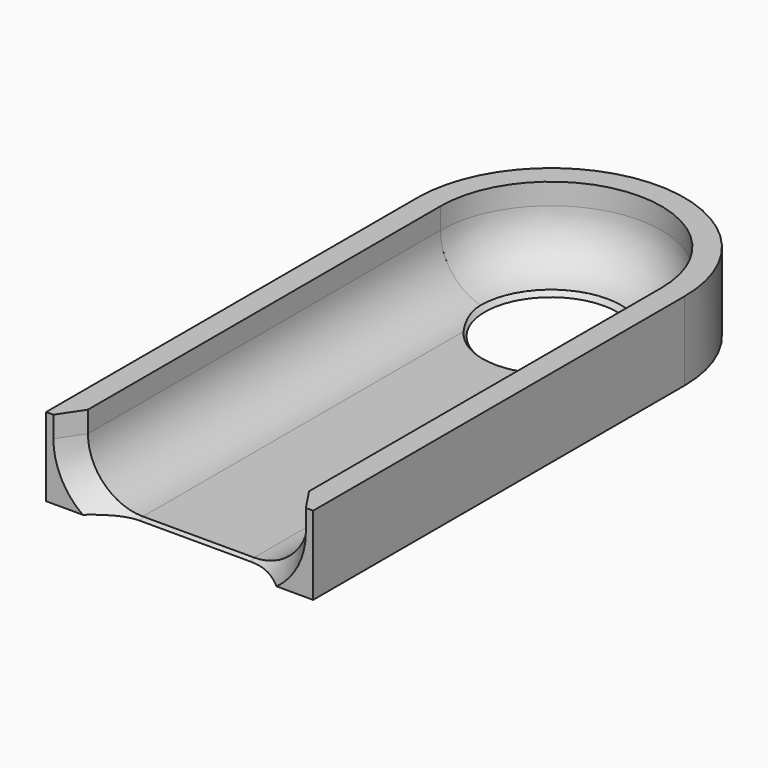
from build123d import *

# Parameters (mm, degrees)
F1_DEPTH     = 25.4
F2_R         = 17.018
F3_DEPTH     = 27.686
F4_R         = 35.7378
F5_DEPTH     = 24.638
F6_R         = 17.7830971004
F7_DEPTH     = 25.4
F8_W         = 71.4756
F8_H         = 155.2468025039
F9_DEPTH     = 24.638
F10_R        = 17.78
F12_T1_DEPTH = 35.9156
F12_T3_DEPTH = 26.5465599919
F12_T6_ANGLE = 90
F12_T8_ANGLE = 90


# Not quite as in the source:
# - a fillet or chamfer that OpenCascade refuses, or shapes differently, is made with other operations: its cross-section is extruded or revolved along the edge and cut away or added


with BuildPart() as f1:
    # F0 (on Top) → F1 (new body)
    with BuildSketch(Plane.XY):
        with BuildLine():
            Line((-43.18, 0), (43.18, 0))
            ThreePointArc((43.18, 0), (0, 43.18), (-43.18, 0))
        make_face()
        with BuildLine():
            ThreePointArc((-43.18, 0), (0, -43.18), (43.18, 0))
            Line((43.18, 0), (-43.18, 0))
        make_face()
    extrude(amount=F1_DEPTH)

    # F2 (on face) → F3 (cut)
    with BuildSketch(Plane.XY):
        Circle(F2_R)
    extrude(amount=F3_DEPTH, mode=Mode.SUBTRACT)

    # F4 (on face) → F5 (cut)
    with BuildSketch(Plane.XY.offset(25.4)):
        Circle(F4_R)
    extrude(amount=-F5_DEPTH, mode=Mode.SUBTRACT)

    # F6
    f6_edges = [f1.edges().sort_by_distance(p)[0] for p in [
        (-35.7378, 0, 0.762),
    ]]
    fillet(f6_edges, radius=F6_R)

    # F0 (on Top) → F7 (join)
    with BuildSketch(Plane.XY):
        with BuildLine():
            Line((43.18, -150.0849872828), (43.18, 0))
            ThreePointArc((43.18, 0), (0, -43.18), (-43.18, 0))
            Line((-43.18, 0), (-43.18, -150.0849872828))
            Line((-43.18, -150.0849872828), (43.18, -150.0849872828))
        make_face()
    extrude(amount=F7_DEPTH)

    # F8 (on face) → F9 (cut)
    with BuildSketch(Plane.XY.offset(25.4)):
        with Locations((0, -77.6234012519)):
            Rectangle(F8_W, F8_H)
    extrude(amount=-F9_DEPTH, mode=Mode.SUBTRACT)

    # F10
    f10_edges = [f1.edges().sort_by_distance(p)[0] for p in [
        (35.7378, -75.042494, 0.762),
        (-35.7378, -75.042494, 0.762),
    ]]
    fillet(f10_edges, radius=F10_R)

    # F11: chamfer of 5.08 on 1 edges, made by hand


with BuildPart() as f11_tool2:
    # F11_s3 → F11_t4 (revolve)
    with BuildSketch(Plane.XZ):
        with BuildLine():
            Line((23.1756307345, 1.8396307345), (15.9403692655, -5.3956307345))
            Line((15.9403692655, -5.3956307345), (15.1783692655, -5.3956307345))
            ThreePointArc((15.1783692655, -5.3956307345), (16.256, -2.3168153673), (16.256, 0.762))
            Line((16.256, 0.762), (17.018, 1.524))
            ThreePointArc((17.018, 1.524), (20.0968153673, 1.524), (23.1756307345, 2.6016307345))
            Line((23.1756307345, 2.6016307345), (23.1756307345, 1.8396307345))
        make_face()
    revolve(axis=Axis((0, 0, 0.762), (0, 0, -1)))

    split(bisect_by=Plane.XZ, keep=Keep.TOP)


with BuildPart() as f1_1:
    add(f1.part)

    # F11_t1: cut F11_tool2
    add(f11_tool2.part, mode=Mode.SUBTRACT)


with BuildPart() as f11_tool7:
    # F11_s8 → F11_t9 (revolve)
    with BuildSketch(Plane.XZ):
        with BuildLine():
            Line((23.1756307345, 1.8396307345), (15.9403692655, -5.3956307345))
            Line((15.9403692655, -5.3956307345), (15.1783692655, -5.3956307345))
            ThreePointArc((15.1783692655, -5.3956307345), (16.256, -2.3168153673), (16.256, 0.762))
            Line((16.256, 0.762), (17.018, 1.524))
            ThreePointArc((17.018, 1.524), (20.0968153673, 1.524), (23.1756307345, 2.6016307345))
            Line((23.1756307345, 2.6016307345), (23.1756307345, 1.8396307345))
        make_face()
    revolve(axis=Axis((0, 0, 0.762), (0, 0, -1)))

    split(bisect_by=Plane.XZ, keep=Keep.BOTTOM)


with BuildPart() as f1_2:
    add(f1_1.part)

    # F11_t6: cut F11_tool7
    add(f11_tool7.part, mode=Mode.SUBTRACT)

    # F12: chamfer of 5.08 x 7.62 on 5 edges, made by hand

    # F12_s2 → F12_t1 (cut)
    with BuildSketch(Plane.YZ.offset(-17.9578)):
        Polygon((-142.4649872828, 0.762), (-150.0849872828, -4.318), (-150.0849872828, 0.762), align=None)
    extrude(amount=F12_T1_DEPTH, mode=Mode.SUBTRACT)

    # F12_s4 → F12_t3 (cut)
    with BuildSketch(Plane.XY.offset(18.542)):
        Polygon((35.7378, -142.4649872828), (40.8178, -150.0849872828), (35.7378, -150.0849872828), align=None)
        Polygon((-35.7378, -142.4649872828), (-40.8178, -150.0849872828), (-35.7378, -150.0849872828), align=None)
    extrude(amount=F12_T3_DEPTH, mode=Mode.SUBTRACT)

    # F12_s5 → F12_t6 (revolve, cut)
    with BuildSketch(Plane.YZ.offset(-17.9578)):
        Polygon((-142.4649872828, 0.762), (-150.0849872828, -4.318), (-150.0849872828, 0.762), align=None)
    revolve(axis=Axis((-17.9578, -150.0849872828, 18.542), (0, 1, 0)), revolution_arc=F12_T6_ANGLE, mode=Mode.SUBTRACT)

    # F12_s7 → F12_t8 (revolve, cut)
    with BuildSketch(Plane.XY.offset(18.542)):
        Polygon((40.8178, -150.0849872828), (35.7378, -142.4649872828), (35.7378, -150.0849872828), align=None)
    revolve(axis=Axis((17.9578, -150.0849872828, 18.542), (0, 1, 0)), revolution_arc=F12_T8_ANGLE, mode=Mode.SUBTRACT)


solid = f1_2.part
